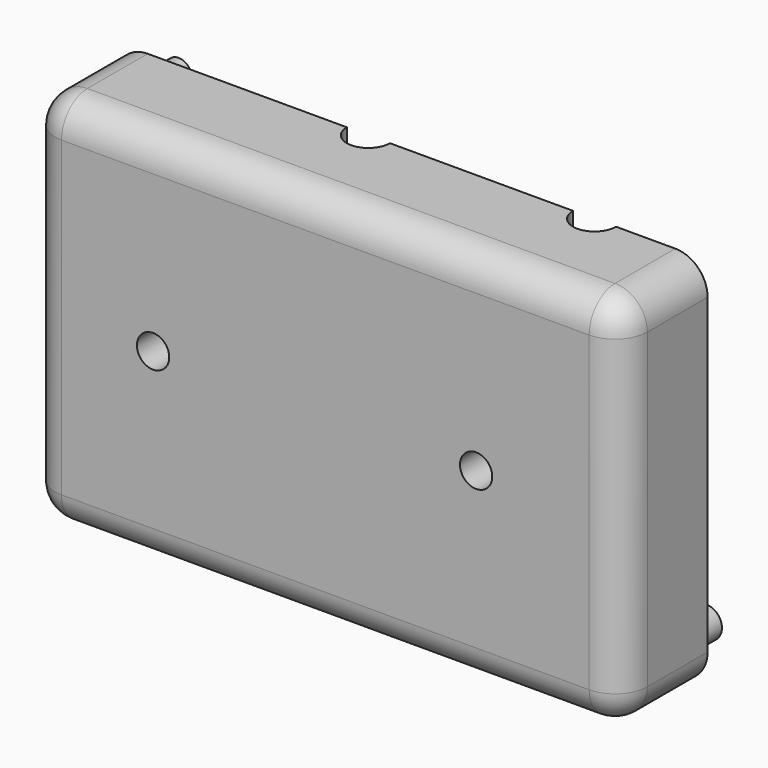
from build123d import *

# Parameters (mm, degrees)
F0_W      = 69.85
F0_H      = 44.45
F1_DEPTH  = 12.7
F2_T      = -6.35
F3_R      = 3.81
F4_R      = 2.54
F5_R      = 1.524
F5_R_2    = 1.8415
F6_DEPTH  = 4.572
F7_R      = 1.905
F8_DEPTH  = 6.35
F9_R      = 2.54
F10_DEPTH = 6.35
F12_DEPTH = 3.175


# Not quite as in the source:
# - a feature names something its author has since deleted; it is built from what else it names


with BuildPart() as f1:
    # F0 (on Front) → F1 (new body)
    with BuildSketch(Plane.XZ):
        Rectangle(F0_W, F0_H)
    extrude(amount=F1_DEPTH)

    # F2
    f2_openings = [f1.faces().sort_by_distance(p)[0] for p in [
        (0, 0, 0),
    ]]
    offset(amount=F2_T, openings=f2_openings)

    # F3
    f3_edges = [f1.edges().sort_by_distance(p)[0] for p in [
        (34.925, -6.35, -22.225),
        (34.925, -12.7, 0),
        (0, -12.7, -22.225),
        (-34.925, -12.7, 0),
        (0, -12.7, 22.225),
        (-34.925, -6.35, 22.225),
        (34.925, -6.35, 22.225),
        (-34.925, -6.35, -22.225),
    ]]
    fillet(f3_edges, radius=F3_R)

    # F4
    f4_edges = [f1.edges().sort_by_distance(p)[0] for p in [
        (-28.575, -6.35, 0),
        (0, -6.35, -15.875),
        (28.575, -6.35, 0),
        (0, -6.35, 15.875),
        (-28.575, -3.175, -15.875),
        (28.575, -3.175, -15.875),
        (28.575, -3.175, 15.875),
        (-28.575, -3.175, 15.875),
    ]]
    fillet(f4_edges, radius=F4_R)

    # F5 (on face) → F6 (join)
    with BuildSketch(Plane(origin=(0, 0, 0), x_dir=(-1, 0, 0), z_dir=(0, 1, 0))):
        with Locations((31.115, 18.415)):
            Circle(F5_R)
        with Locations((-31.115, -18.415)):
            Circle(F5_R_2)
    extrude(amount=F6_DEPTH)

    # F7 (on face) → F8 (cut, through all)
    with BuildSketch(Plane(origin=(0, -6.35, 0), x_dir=(-1, 0, 0), z_dir=(0, 1, 0))):
        with Locations((20.32, 0)):
            Circle(F7_R)
        with Locations((-17.78, 0)):
            Circle(F7_R)
    extrude(amount=-F8_DEPTH, mode=Mode.SUBTRACT)

    # F9 (on face) → F10 (cut, through all)
    with BuildSketch(Plane.XY.offset(22.225)):
        with Locations((-5.08, 0)):
            Circle(F9_R)
        with Locations((21.59, 0)):
            Circle(F9_R)
    extrude(amount=-F10_DEPTH, mode=Mode.SUBTRACT)

    # F11 (on face) → F12 (cut)
    with BuildSketch(Plane(origin=(0, 0, 15.875), x_dir=(1, 0, 0), z_dir=(0, 0, -1))):
        with BuildLine():
            add(Edge.make_bspline(
                [(-8.89, 0), (-8.89, -1.6497783942), (-3.175, -0.8248891971), (2.54, 0), (-3.175, 0.8248891971), (-8.89, 1.6497783942), (-8.89, 0)],
                knots=[0, 0, 0, 2.0943951024, 2.0943951024, 4.1887902048, 4.1887902048, 6.2831853072, 6.2831853072, 6.2831853072], degree=2, weights=[1, 0.5, 1, 0.5, 1, 0.5, 1]))
        make_face()
        with BuildLine():
            add(Edge.make_bspline(
                [(17.78, 0), (17.78, -1.6497783942), (23.495, -0.8248891971), (29.21, 0), (23.495, 0.8248891971), (17.78, 1.6497783942), (17.78, 0)],
                knots=[0, 0, 0, 2.0943951024, 2.0943951024, 4.1887902048, 4.1887902048, 6.2831853072, 6.2831853072, 6.2831853072], degree=2, weights=[1, 0.5, 1, 0.5, 1, 0.5, 1]))
        make_face()
    extrude(amount=-F12_DEPTH, mode=Mode.SUBTRACT)


solid = f1.part
